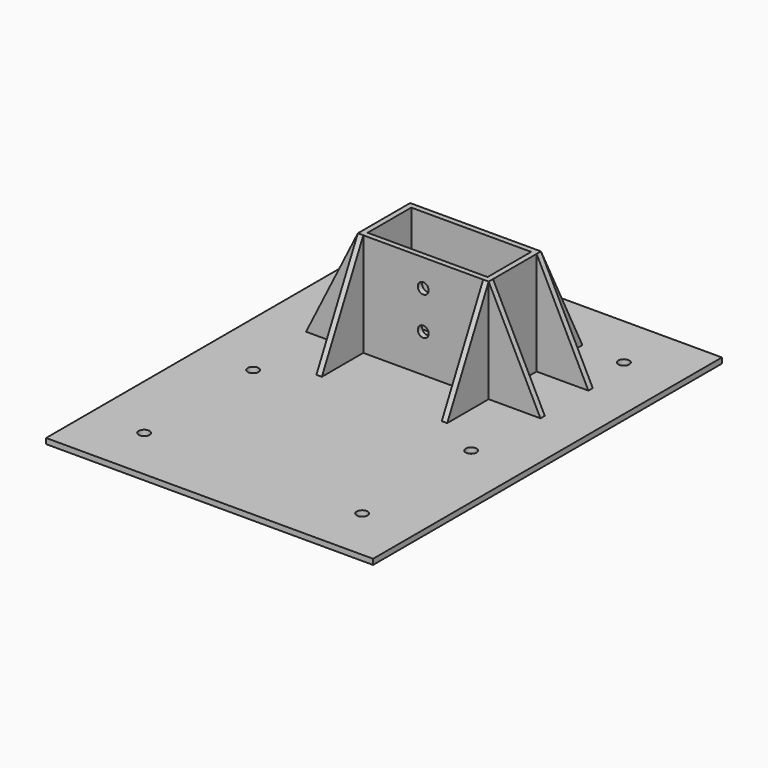
from build123d import *

# Parameters (mm, degrees)
F0_W         = 5
F0_H         = 50
F0_H_2       = 5
F0_W_2       = 50
F0_W_3       = 110
F1_DEPTH     = 100
F0_W_4       = 300
F0_H_3       = 400
F2_DEPTH     = 5
F3_T4_DEPTH  = 522.9657747574
F3_T9_DEPTH  = 522.9657747574
F3_T14_DEPTH = 522.9657747574
F3_T19_DEPTH = 522.9657747574
F3_T24_DEPTH = 522.9657747574
F3_T29_DEPTH = 522.9657747574
F3_T34_DEPTH = 522.9657747574
F3_T39_DEPTH = 522.9657747574
F3_T44_DEPTH = 522.9657747574
F6_D         = 10
F6_DEPTH     = 20
F6_TIP       = 3.0043030951
F7_D         = 10
F7_DEPTH     = 20
F7_TIP       = 3.0043030951


# Not quite as in the source:
# - a fillet or chamfer that OpenCascade refuses, or shapes differently, is made with other operations: its cross-section is extruded or revolved along the edge and cut away or added


with BuildPart() as f1:
    # F0 (on Top) → F1 (new body)
    with BuildSketch(Plane.XY):
        with Locations((-57.5, 130)):
            Rectangle(F0_W, F0_H)
        with Locations((-57.5, 20)):
            Rectangle(F0_W, F0_H)
        with Locations((-57.5, 102.5)):
            Rectangle(F0_W, F0_H_2)
        with Locations((57.5, 102.5)):
            Rectangle(F0_W, F0_H_2)
        with Locations((-85, 47.5)):
            Rectangle(F0_W_2, F0_H_2)
        with Locations((-85, 102.5)):
            Rectangle(F0_W_2, F0_H_2)
        Polygon((-55, 105), (-55, 100), (55, 100), (55, 105), (2.5, 105), (-2.5, 105), align=None)
        with Locations((57.5, 47.5)):
            Rectangle(F0_W, F0_H_2)
        with Locations((57.5, 75)):
            Rectangle(F0_W, F0_H)
        with Locations((0, 47.5)):
            Rectangle(F0_W_3, F0_H_2)
        with Locations((57.5, 130)):
            Rectangle(F0_W, F0_H)
        with Locations((85, 102.5)):
            Rectangle(F0_W_2, F0_H_2)
        with Locations((-57.5, 47.5)):
            Rectangle(F0_W, F0_H_2)
        with Locations((85, 47.5)):
            Rectangle(F0_W_2, F0_H_2)
        with Locations((-57.5, 75)):
            Rectangle(F0_W, F0_H)
        with Locations((57.5, 20)):
            Rectangle(F0_W, F0_H)
        with Locations((0, 130)):
            Rectangle(F0_W, F0_H)
    extrude(amount=F1_DEPTH)

    # F0 (on Top) → F2 (join)
    with BuildSketch(Plane.XY):
        Rectangle(F0_W_4, F0_H_3)
        Polygon((55, 45), (-55, 45), (-55, -5), (-60, -5), (-60, 45), (-110, 45), (-110, 50), (-60, 50), (-60, 100), (-110, 100), (-110, 105), (-60, 105), (-60, 155), (-55, 155), (-55, 105), (-2.5, 105), (-2.5, 155), (2.5, 155), (2.5, 105), (55, 105), (55, 155), (60, 155), (60, 105), (110, 105), (110, 100), (60, 100), (60, 50), (110, 50), (110, 45), (60, 45), (60, -5), (55, -5), align=None, mode=Mode.SUBTRACT)
        with Locations((0, 75)):
            Rectangle(F0_W_3, F0_H)
    extrude(amount=F2_DEPTH)

    # F3: chamfer of 50 x 100 on 9 edges, made by hand


with BuildPart() as f3_tool2:
    # F3_s3 → F3_t4 (new body)
    with BuildSketch(Plane.XZ.offset(213.9828873787)):
        Polygon((60, 100), (110, 0), (110, 100), align=None)
    extrude(amount=-F3_T4_DEPTH)

    split(bisect_by=Plane.XY.offset(5), keep=Keep.TOP)


with BuildPart() as f1_1:
    add(f1.part)

    # F3_t1: cut F3_tool2
    add(f3_tool2.part, mode=Mode.SUBTRACT)


with BuildPart() as f3_tool7:
    # F3_s8 → F3_t9 (new body)
    with BuildSketch(Plane.XZ.offset(158.9828873787)):
        Polygon((60, 100), (110, 0), (110, 100), align=None)
    extrude(amount=-F3_T9_DEPTH)

    split(bisect_by=Plane.XY.offset(5), keep=Keep.TOP)


with BuildPart() as f1_2:
    add(f1_1.part)

    # F3_t6: cut F3_tool7
    add(f3_tool7.part, mode=Mode.SUBTRACT)


with BuildPart() as f3_tool12:
    # F3_s13 → F3_t14 (new body)
    with BuildSketch(Plane.YZ.offset(-203.9828873787)):
        Polygon((45, 100), (-5, 0), (-5, 100), align=None)
    extrude(amount=F3_T14_DEPTH)

    split(bisect_by=Plane.XY.offset(5), keep=Keep.TOP)


with BuildPart() as f1_3:
    add(f1_2.part)

    # F3_t11: cut F3_tool12
    add(f3_tool12.part, mode=Mode.SUBTRACT)


with BuildPart() as f3_tool17:
    # F3_s18 → F3_t19 (new body)
    with BuildSketch(Plane.YZ.offset(318.9828873787)):
        Polygon((105, 100), (155, 0), (155, 100), align=None)
    extrude(amount=-F3_T19_DEPTH)

    split(bisect_by=Plane.XY.offset(5), keep=Keep.TOP)


with BuildPart() as f1_4:
    add(f1_3.part)

    # F3_t16: cut F3_tool17
    add(f3_tool17.part, mode=Mode.SUBTRACT)


with BuildPart() as f3_tool22:
    # F3_s23 → F3_t24 (new body)
    with BuildSketch(Plane.YZ.offset(-318.9828873787)):
        Polygon((45, 100), (-5, 0), (-5, 100), align=None)
    extrude(amount=F3_T24_DEPTH)

    split(bisect_by=Plane.XY.offset(5), keep=Keep.TOP)


with BuildPart() as f1_5:
    add(f1_4.part)

    # F3_t21: cut F3_tool22
    add(f3_tool22.part, mode=Mode.SUBTRACT)


with BuildPart() as f3_tool27:
    # F3_s28 → F3_t29 (new body)
    with BuildSketch(Plane.XZ.offset(-308.9828873787)):
        Polygon((-60, 100), (-110, 0), (-110, 100), align=None)
    extrude(amount=F3_T29_DEPTH)

    split(bisect_by=Plane.XY.offset(5), keep=Keep.TOP)


with BuildPart() as f1_6:
    add(f1_5.part)

    # F3_t26: cut F3_tool27
    add(f3_tool27.part, mode=Mode.SUBTRACT)


with BuildPart() as f3_tool32:
    # F3_s33 → F3_t34 (new body)
    with BuildSketch(Plane.XZ.offset(-363.9828873787)):
        Polygon((-60, 100), (-110, 0), (-110, 100), align=None)
    extrude(amount=F3_T34_DEPTH)

    split(bisect_by=Plane.XY.offset(5), keep=Keep.TOP)


with BuildPart() as f1_7:
    add(f1_6.part)

    # F3_t31: cut F3_tool32
    add(f3_tool32.part, mode=Mode.SUBTRACT)


with BuildPart() as f3_tool37:
    # F3_s38 → F3_t39 (new body)
    with BuildSketch(Plane.YZ.offset(203.9828873787)):
        Polygon((155, 0), (105, 100), (155, 100), align=None)
    extrude(amount=-F3_T39_DEPTH)

    split(bisect_by=Plane.XY.offset(5), keep=Keep.TOP)


with BuildPart() as f1_8:
    add(f1_7.part)

    # F3_t36: cut F3_tool37
    add(f3_tool37.part, mode=Mode.SUBTRACT)


with BuildPart() as f3_tool42:
    # F3_s43 → F3_t44 (new body)
    with BuildSketch(Plane.YZ.offset(261.4828873787)):
        Polygon((105, 100), (155, 0), (155, 100), align=None)
    extrude(amount=-F3_T44_DEPTH)

    split(bisect_by=Plane.XY.offset(5), keep=Keep.TOP)


with BuildPart() as f1_9:
    add(f1_8.part)

    # F3_t41: cut F3_tool42
    add(f3_tool42.part, mode=Mode.SUBTRACT)

    # F6
    with Locations(Plane.XZ.offset(-44.9998)):
        with Locations((0, 40), (0, 75)):
            Hole(F6_D / 2, depth=F6_DEPTH)
            with Locations((0, 0, -(F6_DEPTH + F6_TIP / 2))):  # 118° drill point
                Cone(0, F6_D / 2, F6_TIP, mode=Mode.SUBTRACT)

    # F7
    with Locations(Plane(origin=(0, 0, 0), x_dir=(1, 0, 0), z_dir=(0, 0, -1))):
        with Locations((-100, 25), (-100, -150), (100, -150), (100, 25), (100, 150), (-100, 150)):
            Hole(F7_D / 2, depth=F7_DEPTH)
            with Locations((0, 0, -(F7_DEPTH + F7_TIP / 2))):  # 118° drill point
                Cone(0, F7_D / 2, F7_TIP, mode=Mode.SUBTRACT)


solid = f1_9.part
